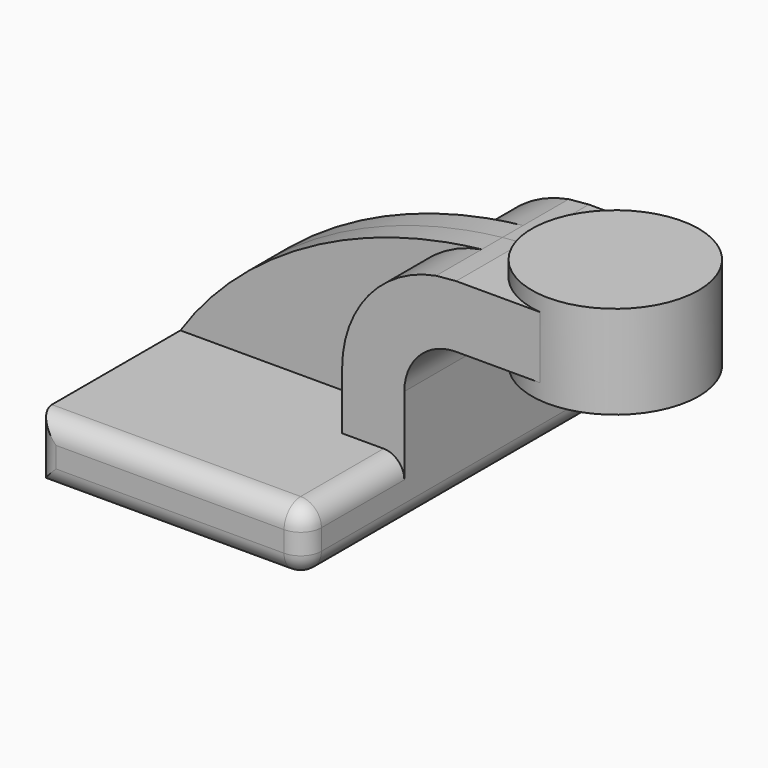
from build123d import *

# Parameters (mm, degrees)
F1_DEPTH = 63.5
F2_DEPTH = 7.9375
F0_W     = 25.2498040683
F0_H     = 19.05
F3_DEPTH = 25.4
F5_R     = 6.35


# Not quite as in the source:
# - a feature names something its author has since deleted; it is built from what else it names


with BuildPart() as f1:
    # F0 (on Front) → F1 (new body, symmetric)
    with BuildSketch(Plane.XZ):
        Polygon((-41.275, -9.525), (41.275, -9.525), (41.275, 9.525), (22.225, 9.525), (-41.275, 9.525), align=None)
    extrude(amount=F1_DEPTH, both=True)

    # F0 (on Front) → F2 (join, symmetric)
    with BuildSketch(Plane.XZ):
        with BuildLine():
            add(Edge.make_bspline(
                [(-41.275, 9.525), (-23.4670489943, 36.4343195367), (10.3939996221, 56.9389145817), (51.0054120889, 61.3804219947)],
                knots=[0, 0, 0, 0, 106.1920094682, 106.1920094682, 106.1920094682, 106.1920094682], degree=3))
            Line((-41.275, 9.525), (22.225, 9.525))
            Line((22.225, 9.525), (22.225, 27.0002))
            ThreePointArc((22.225, 27.0002), (30.3698267575, 49.4184502908), (51.0054120889, 61.3804219947))
        make_face()
    extrude(amount=F2_DEPTH, both=True)

    # F0 (on Front) → F3 (join, symmetric)
    with BuildSketch(Plane.XZ):
        with BuildLine():
            Line((22.225, 9.525), (41.275, 9.525))
            Line((41.275, 9.525), (41.275, 27.0002))
            ThreePointArc((41.275, 27.0002), (45.9246798487, 38.2255201513), (57.15, 42.8752))
            Line((57.15, 42.8752), (60.325, 42.8752))
            Line((60.325, 42.8752), (60.325, 61.9252))
            Line((60.325, 61.9252), (57.15, 61.9252))
            add(Edge.make_bspline(
                [(51.0054120889, 61.3804219947), (53.0371017984, 61.6026197553), (55.0856860239, 61.7846155213), (57.15, 61.9252)],
                knots=[106.1920094682, 106.1920094682, 106.1920094682, 106.1920094682, 111.5045361635, 111.5045361635, 111.5045361635, 111.5045361635], degree=3))
            ThreePointArc((51.0054120889, 61.3804219947), (30.3698267575, 49.4184502908), (22.225, 27.0002))
            Line((22.225, 27.0002), (22.225, 9.525))
        make_face()
        with Locations((72.9499020342, 52.4002)):
            Rectangle(F0_W, F0_H)
    extrude(amount=F3_DEPTH, both=True)

    # F0 (on Front) → F4 (revolve)
    with BuildSketch(Plane.XZ):
        Polygon((85.5748040683, 61.9252), (85.5748040683, 42.8752), (85.5748040683, 38.1), (111.125, 38.1), (111.125, 66.675), (85.5748040683, 66.675), align=None)
    revolve(axis=Axis((85.5748040683, 0, 52.3875), (0, 0, -1)))

    # F5
    f5_edges = [f1.edges().sort_by_distance(p)[0] for p in [
        (41.275, -63.5, 0),
        (-41.275, -63.5, 0),
        (0, -63.5, 9.525),
        (41.275, 0, -9.525),
        (0, -63.5, -9.525),
        (41.275, -44.45, 9.525),
        (-41.275, 63.5, 0),
        (41.275, 63.5, 0),
    ]]
    fillet(f5_edges, radius=F5_R)


solid = f1.part
